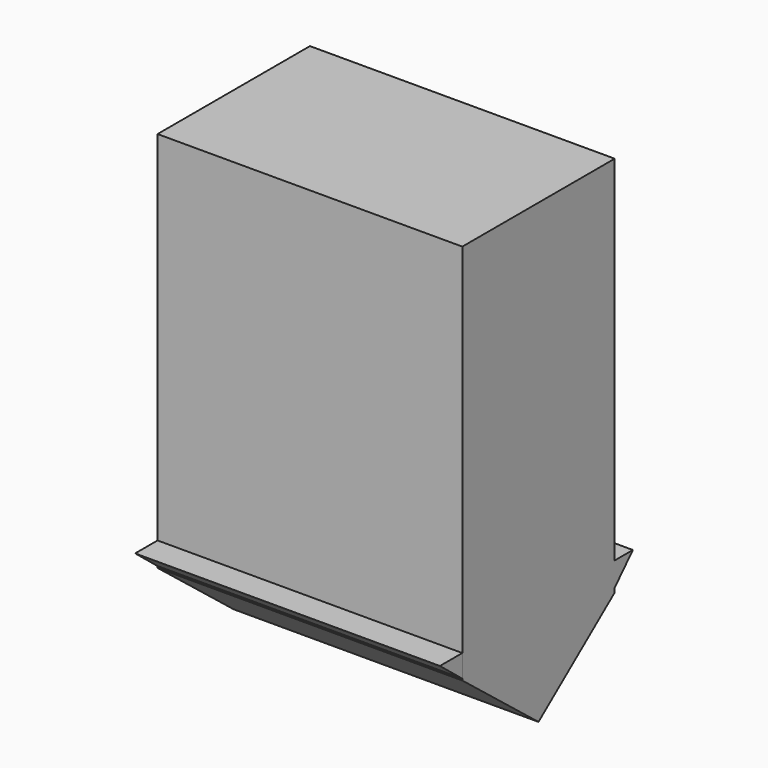
from build123d import *

# Parameters (mm, degrees)
F0_W      = 25.4
F0_H      = 38.1
F1_DEPTH  = 15.875
F3_DEPTH  = 50.8
F5_DEPTH  = 50.8
F7_DEPTH  = 25.4
F10_DEPTH = 25.4


# Not quite as in the source:
# - a feature names something its author has since deleted; it is built from what else it names


with BuildPart() as f1:
    # F0 (on Front) → F1 (new body)
    with BuildSketch(Plane.XZ):
        Rectangle(F0_W, F0_H)
    extrude(amount=F1_DEPTH)

    # F2 (on face) → F3 (cut)
    with BuildSketch(Plane(origin=(-12.7, 0, 0), x_dir=(0, -1, 0), z_dir=(-1, 0, 0))):
        Polygon((15.875, -12.7851702273), (7.9375, -19.05), (15.875, -19.05), align=None)
    extrude(amount=-F3_DEPTH, mode=Mode.SUBTRACT)

    # F4 (on face) → F5 (cut)
    with BuildSketch(Plane(origin=(-12.7, 0, 0), x_dir=(0, -1, 0), z_dir=(-1, 0, 0))):
        Polygon((7.9375, -19.05), (0, -12.7851702273), (0, -19.05), align=None)
    extrude(amount=-F5_DEPTH, mode=Mode.SUBTRACT)

    # F6 (on face) → F7 (join)
    with BuildSketch(Plane(origin=(-12.7, 0, 0), x_dir=(0, -1, 0), z_dir=(-1, 0, 0))):
        Polygon((0, -12.4311430186), (0, -10.4295834899), (-1.8933862448, -10.4295834899), align=None)
    extrude(amount=-F7_DEPTH)


with BuildPart() as f10:
    # F9 (on face) → F10 (new body)
    with BuildSketch(Plane(origin=(-12.7, 0, 0), x_dir=(0, -1, 0), z_dir=(-1, 0, 0))):
        Polygon((18.2110549376, -10.7685425392), (15.875, -10.7685425392), (15.875, -12.64857003), align=None)
    extrude(amount=-F10_DEPTH)


solid = Compound([f1.part, f10.part])
